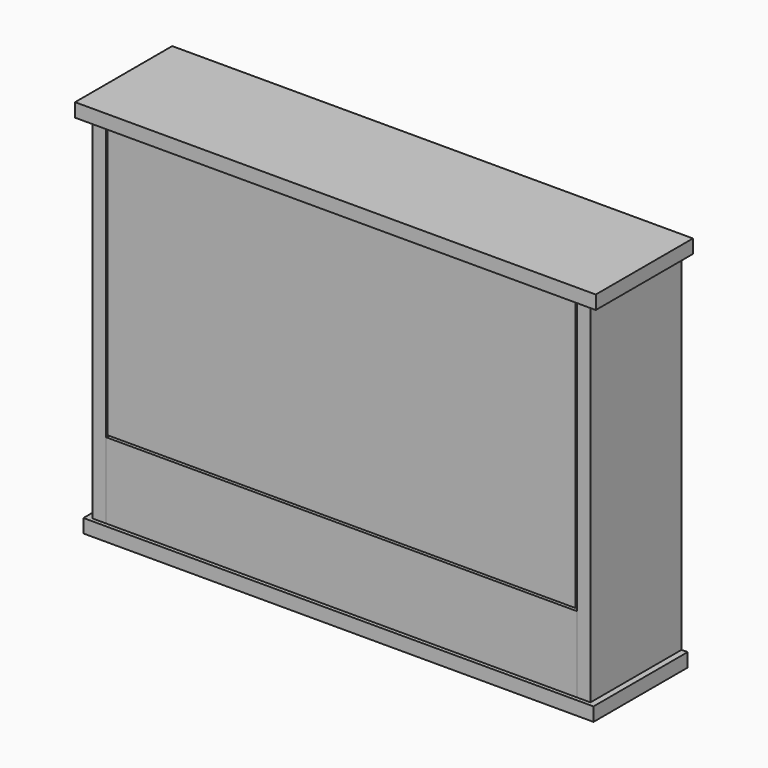
from build123d import *

# Parameters (mm, degrees)
F2_DEPTH = 150
F3_DEPTH = 155
F4_START = 132
F1_W     = 620
F1_H     = 100
F4_DEPTH = 18
F5_DEPTH = 160
F6_START = 132
F1_W_2   = 616
F1_H_2   = 359
F6_DEPTH = 18
F7_W     = 620
F7_H     = 80
F8_DEPTH = 18


# Not quite as in the source:
# - a feature of the source that left no trace in its solid (it failed there, or was rolled back) is left out


with BuildPart() as f2:
    # F1 (on Front) → F2 (new body)
    with BuildSketch(Plane.XZ):
        Polygon((-310, 118), (-310, 482), (-328, 482), (-328, 18), (-310, 18), align=None)
    extrude(amount=F2_DEPTH)


with BuildPart() as f2b:
    # F1 (on Front) → F2, piece 2 (new body)
    with BuildSketch(Plane.XZ):
        Polygon((328, 482), (310, 482), (310, 118), (310, 18), (328, 18), align=None)
    extrude(amount=F2_DEPTH)


with BuildPart() as f3:
    # F1 (on Front) → F3 (new body, through all)
    with BuildSketch(Plane.XZ):
        Polygon((310, 18), (-310, 18), (-328, 18), (-336, 18), (-336, 0), (-328, 0), (328, 0), (336, 0), (336, 18), (328, 18), align=None)
    extrude(amount=F3_DEPTH)


with BuildPart() as f4:
    # F1 (on Front) → F4 (new body)
    with BuildSketch(Plane.XZ.offset(F4_START)):
        with Locations((0, 68)):
            Rectangle(F1_W, F1_H)
    extrude(amount=F4_DEPTH)


with BuildPart() as f5:
    # F1 (on Front) → F5 (new body, through all)
    with BuildSketch(Plane.XZ):
        Polygon((-328, 482), (-310, 482), (310, 482), (328, 482), (343, 482), (343, 500), (328, 500), (-328, 500), (-343, 500), (-343, 482), align=None)
    extrude(amount=F5_DEPTH)


with BuildPart() as f6:
    # F1 (on Front) → F6 (new body)
    with BuildSketch(Plane.XZ.offset(F6_START)):
        with Locations((0, 300.5)):
            Rectangle(F1_W_2, F1_H_2)
    extrude(amount=F6_DEPTH)


with BuildPart() as f8:
    # F7 (on face) → F8 (new body)
    with BuildSketch(Plane.XZ):
        with Locations((0, 442)):
            Rectangle(F7_W, F7_H)
    extrude(amount=F8_DEPTH)


solid = Compound([f2.part, f2b.part, f3.part, f4.part, f5.part, f6.part, f8.part])
